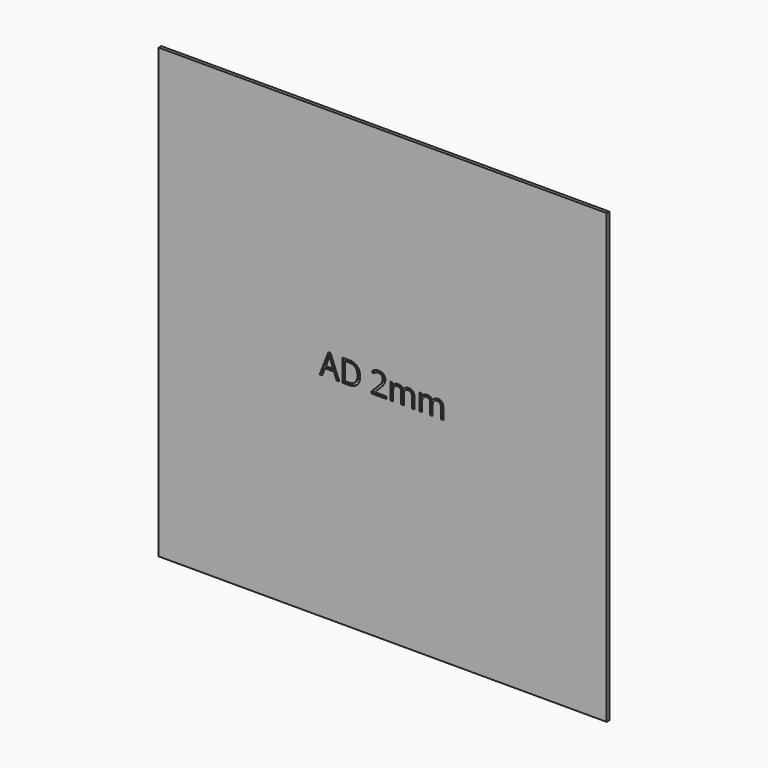
from build123d import *

# Parameters (mm, degrees)
F0_W         = 276.5
F0_H         = 276.5
F1_DEPTH     = 2
F2_TEXT_SIZE = 19.2192512461
F3_DEPTH     = 1


# Not quite as in the source:
# - Text() gives the source's letters only with a copy of the font that has no kerning and outlines rounded to 1/6400 em; it was checked with that copy


with BuildPart() as f1:
    # F0 (on Front) → F1 (new body)
    with BuildSketch(Plane.XZ):
        with Locations((138.25, 138.25)):
            Rectangle(F0_W, F0_H)
    extrude(amount=F1_DEPTH)

    # F2 (on face) → F3 (cut)
    with BuildSketch(Plane.XZ.offset(2)):
        with Locations((99.3246939033, 131.2344977632)):
            Text('AD 2mm', F2_TEXT_SIZE, font='Open Sans', text_align=(TextAlign.LEFT, TextAlign.BOTTOM))
    extrude(amount=-F3_DEPTH, mode=Mode.SUBTRACT)


solid = f1.part
